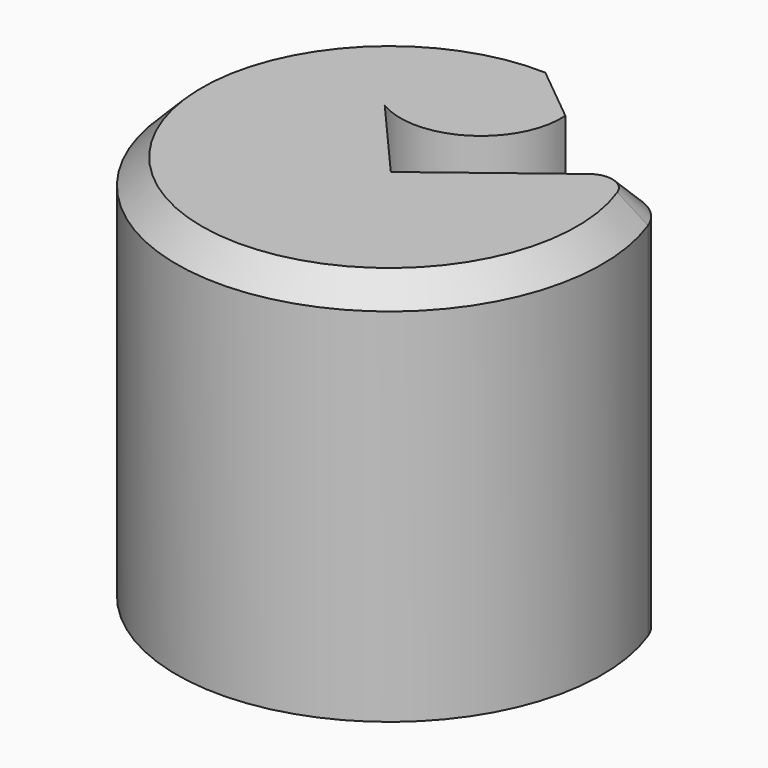
from build123d import *

# Parameters (mm, degrees)
F1_DEPTH    = 77.978
F2_R        = 9.8113639175
F3_T1_DEPTH = 141.3502926448
F4_SIZE     = 5.08


# Not quite as in the source:
# - a fillet or chamfer that OpenCascade refuses, or shapes differently, is made with other operations: its cross-section is extruded or revolved along the edge and cut away or added


with BuildPart() as f1:
    # F0 (on Top) → F1 (new body)
    with BuildSketch(Plane.XY):
        with BuildLine():
            Line((-7.4381157756, 43.2214848697), (-39.8039706051, 38.5977886617))
            ThreePointArc((-39.8039706051, 38.5977886617), (-21.172854192, -38.7924441896), (19.2988961935, 29.7524612397))
            Line((19.2988961935, 29.7524612397), (-14.8171193926, 3.6754181444))
            Line((-14.8171193926, 3.6754181444), (-26.3349507004, 16.8865323067))
            ThreePointArc((-26.3349507004, 16.8865323067), (-4.9953492686, 21.5214038686), (-7.4381157756, 43.2214848697))
        make_face()
    extrude(amount=F1_DEPTH)

    # F2
    f2_edges = [f1.edges().sort_by_distance(p)[0] for p in [
        (19.298896, 29.752461, 38.989),
    ]]
    fillet(f2_edges, radius=F2_R)

    # F3: chamfer of 5.08 on 1 edges, made by hand

    # F3_s2 → F3_t1 (cut)
    with BuildSketch(Plane.XY.offset(-31.6861463224)):
        with BuildLine():
            Line((-14.6495810062, 42.3422516773), (-1.8120830861, 31.8641235926))
            Line((-1.8120830861, 31.8641235926), (-1.7106647042, 31.8701958104))
            ThreePointArc((-1.7106647042, 31.8701958104), (-3.4500397911, 38.1062153929), (-7.3708029252, 43.2975870391))
            Line((-7.3708029252, 43.2975870391), (-7.4524841935, 43.3220637371))
            ThreePointArc((-7.4524841935, 43.3220637371), (-11.0476484326, 42.8084685502), (-14.663949424, 42.4428305447))
            Line((-14.663949424, 42.4428305447), (-14.6495810062, 42.3422516773))
        make_face()
    extrude(amount=F3_T1_DEPTH, mode=Mode.SUBTRACT)

    # F4
    f4_edges = [f1.edges().sort_by_distance(p)[0] for p in [
        (-27.46138, -37.361606, 77.978),
        (19.021994, 24.517514, 77.978),
        (-2.246992, 13.283567, 77.978),
    ]]
    chamfer(f4_edges, length=F4_SIZE)


solid = f1.part
